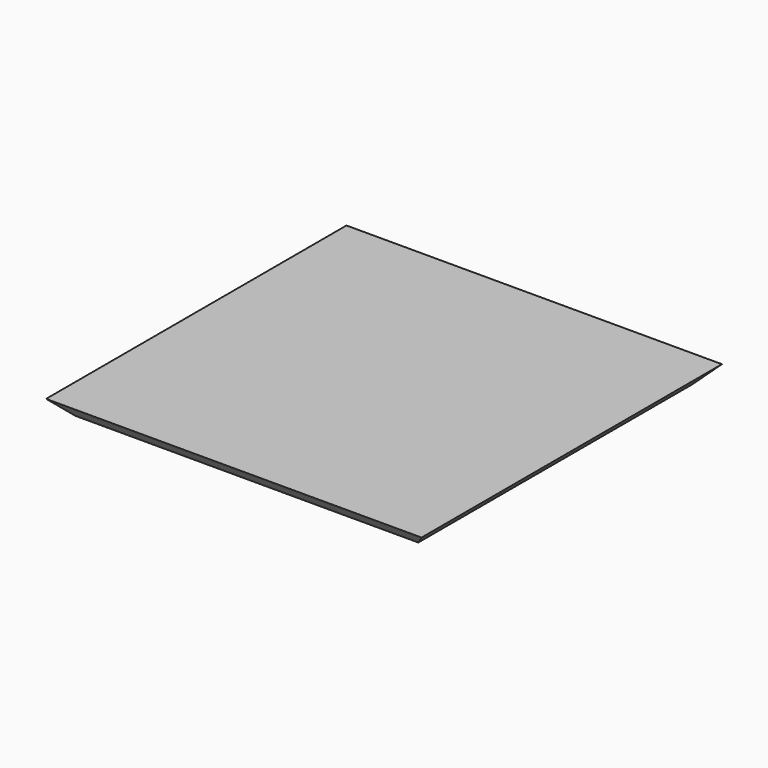
from build123d import *

# Parameters (mm, degrees)
F0_W     = 584.2
F0_H     = 584.2
F1_DEPTH = 25.4
F2_SIZE  = 25.39999


# Not quite as in the source:
# - a fillet or chamfer is up to 0.001 mm smaller than in the source, because OpenCascade refuses the exact size


with BuildPart() as f1:
    # F0 (on Top) → F1 (new body)
    with BuildSketch(Plane.XY):
        Rectangle(F0_W, F0_H)
    extrude(amount=F1_DEPTH)

    # F2 (size 25.4 in the source; OpenCascade refuses exactly that, so slightly less here)
    f2_edges = [f1.edges().sort_by_distance(p)[0] for p in [
        (0, 292.1, 0),
        (-292.1, 0, 0),
        (0, -292.1, 0),
        (292.1, 0, 0),
    ]]
    chamfer(f2_edges, length=F2_SIZE)


solid = f1.part
